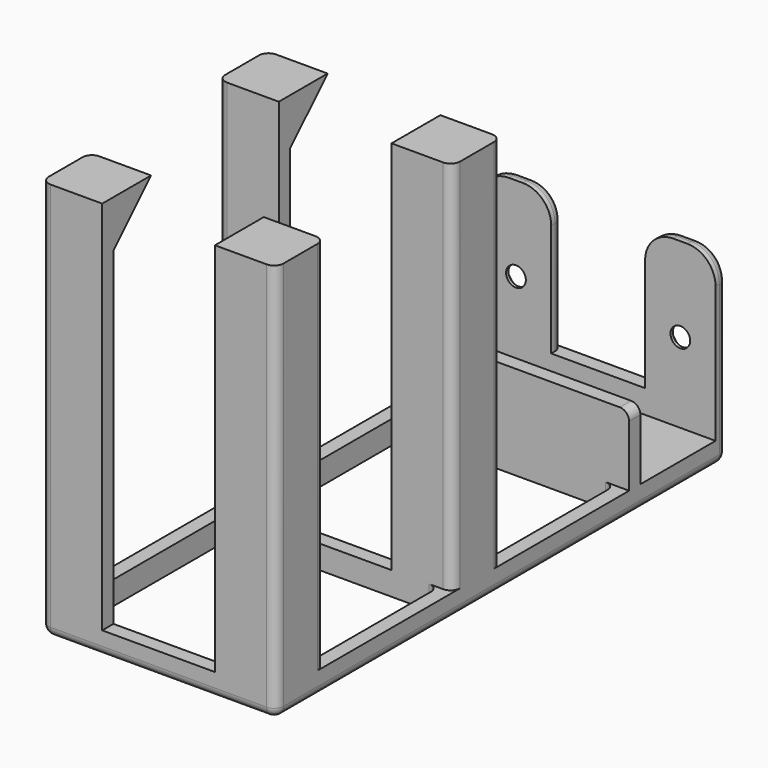
from build123d import *

# Parameters (mm, degrees)
F0_W            = 50
F0_H            = 120
F0_W_2          = 44
F0_H_2          = 44
F1_DEPTH        = 5
F2_W            = 50
F2_H            = 3
F3_DEPTH        = 35
F4_DEPTH        = 15
F5_DEPTH        = 80
F6_W            = 10
F6_H            = 10
F7_W            = 10
F7_H            = 10
F8_DEPTH        = 10
F9_SIZE         = 9.99999
F10_W           = 20
F10_H           = 30
F11_DEPTH       = 3
F12_R           = 6
F13_F1_R        = 2
F13_F2_R        = 2
F13_F3_R        = 2
F13_F4_R        = 2
F13_F5_R        = 2
F13_F6_R        = 2
F13_F7_R        = 2
F13_F8_R        = 2
F13_F9_R        = 2
F13_F10_R       = 2
F13_F11_R       = 2
F13_F12_R       = 2
F13_F13_R       = 2
F13_F14_R       = 2
F13_F15_R       = 2
F13_F16_R       = 2
F13_F17_R       = 2
F13_F18_R       = 2
F13_F19_R       = 2
F13_F20_R       = 2
F15_D           = 4.2
F15_DEPTH       = 12
F15_CSINK_D     = 8.96
F15_CSINK_ANGLE = 90
F15_TIP         = 1.2618073


# Not quite as in the source:
# - a fillet or chamfer is up to 0.001 mm smaller than in the source, because OpenCascade refuses the exact size


with BuildPart() as f1:
    # F0 (on Top) → F1 (new body)
    with BuildSketch(Plane.XY):
        with Locations((0, 11.5)):
            Rectangle(F0_W, F0_H)
        with Locations((0, -23.5)):
            Rectangle(F0_W_2, F0_H_2, mode=Mode.SUBTRACT)
        with Locations((0, 23.5)):
            Rectangle(F0_W_2, F0_H_2, mode=Mode.SUBTRACT)
    extrude(amount=F1_DEPTH)

    # F2 (on face) → F3 (join)
    with BuildSketch(Plane.XY.offset(5)):
        with Locations((0, 70)):
            Rectangle(F2_W, F2_H)
    extrude(amount=F3_DEPTH)

    # F2 (on face) → F4 (join)
    with BuildSketch(Plane.XY.offset(5)):
        Polygon((25, 48.5), (-25, 48.5), (-25, 45.5), (-22, 45.5), (22, 45.5), (25, 45.5), align=None)
    extrude(amount=F4_DEPTH)

    # F2 (on face) → F5 (join)
    with BuildSketch(Plane.XY.offset(5)):
        Polygon((-22, 11.5), (-25, 11.5), (-25, -1.5), (-22, -1.5), (-12, -1.5), (-12, 1.5), (-22, 1.5), align=None)
        Polygon((25, -1.5), (25, 11.5), (22, 11.5), (22, 1.5), (12, 1.5), (12, -1.5), (22, -1.5), align=None)
        Polygon((-22, -35.5), (-25, -35.5), (-25, -48.5), (-12, -48.5), (-12, -45.5), (-22, -45.5), align=None)
        Polygon((25, -48.5), (25, -35.5), (22, -35.5), (22, -45.5), (12, -45.5), (12, -48.5), align=None)
    extrude(amount=F5_DEPTH)

    # F6 (on face) + F7 (on face) → F8 (join)
    with BuildSketch(Plane(origin=(0, 1.5, 0), x_dir=(-1, 0, 0), z_dir=(0, 1, 0))):
        with Locations((-17, 80)):
            Rectangle(F6_W, F6_H)
        with Locations((17, 80)):
            Rectangle(F6_W, F6_H)
    with BuildSketch(Plane(origin=(0, -45.5, 0), x_dir=(-1, 0, 0), z_dir=(0, 1, 0))):
        with Locations((17, 80)):
            Rectangle(F7_W, F7_H)
        with Locations((-17, 80)):
            Rectangle(F7_W, F7_H)
    extrude(amount=F8_DEPTH)

    # F9 (size 10 in the source; OpenCascade refuses exactly that, so slightly less here)
    f9_edges = [f1.edges().sort_by_distance(p)[0] for p in [
        (-17, 11.5, 75),
        (-17, -35.5, 75),
        (17, 11.5, 75),
        (17, -35.5, 75),
    ]]
    chamfer(f9_edges, length=F9_SIZE)

    # F10 (on face) → F11 (cut, through all)
    with BuildSketch(Plane(origin=(0, 71.5, 0), x_dir=(-1, 0, 0), z_dir=(0, 1, 0))):
        with Locations((0, 25)):
            Rectangle(F10_W, F10_H)
    extrude(amount=-F11_DEPTH, mode=Mode.SUBTRACT)

    # F12
    f12_edges = [f1.edges().sort_by_distance(p)[0] for p in [
        (25, 70, 40),
        (10, 70, 40),
        (-10, 70, 40),
        (-25, 70, 40),
    ]]
    fillet(f12_edges, radius=F12_R)

    # F13: fillet of radius 2 on 36 edges, made by hand

    # F13_f1
    f13_f1_edges = [f1.edges().sort_by_distance(p)[0] for p in [
        (25, 71.5, 17),
        (23.2426406871, 71.5, 38.2426406871),
        (17.5, 71.5, 40),
        (11.7573593129, 71.5, 38.2426406871),
        (10, 71.5, 22),
    ]]
    fillet(f13_f1_edges, radius=F13_F1_R)

    # F13_f2
    f13_f2_edges = [f1.edges().sort_by_distance(p)[0] for p in [
        (25, 10.5, 0),
    ]]
    fillet(f13_f2_edges, radius=F13_F2_R)

    # F13_f3
    f13_f3_edges = [f1.edges().sort_by_distance(p)[0] for p in [
        (25, 47, 20),
    ]]
    fillet(f13_f3_edges, radius=F13_F3_R)

    # F13_f4
    f13_f4_edges = [f1.edges().sort_by_distance(p)[0] for p in [
        (25, -48.5, 43.5),
    ]]
    fillet(f13_f4_edges, radius=F13_F4_R)

    # F13_f5
    f13_f5_edges = [f1.edges().sort_by_distance(p)[0] for p in [
        (25, -35.5, 45),
    ]]
    fillet(f13_f5_edges, radius=F13_F5_R)

    # F13_f6
    f13_f6_edges = [f1.edges().sort_by_distance(p)[0] for p in [
        (25, 11.5, 45),
    ]]
    fillet(f13_f6_edges, radius=F13_F6_R)

    # F13_f7
    f13_f7_edges = [f1.edges().sort_by_distance(p)[0] for p in [
        (25, -1.5, 45),
    ]]
    fillet(f13_f7_edges, radius=F13_F7_R)

    # F13_f8
    f13_f8_edges = [f1.edges().sort_by_distance(p)[0] for p in [
        (-25, 71.5, 18),
        (-23.2426406871, 71.5, 38.2426406871),
        (-17.5, 71.5, 40),
        (-11.7573593129, 71.5, 38.2426406871),
        (-10, 71.5, 22),
    ]]
    fillet(f13_f8_edges, radius=F13_F8_R)

    # F13_f9
    f13_f9_edges = [f1.edges().sort_by_distance(p)[0] for p in [
        (-25, -35.5, 45),
    ]]
    fillet(f13_f9_edges, radius=F13_F9_R)

    # F13_f10
    f13_f10_edges = [f1.edges().sort_by_distance(p)[0] for p in [
        (-25, 47, 20),
    ]]
    fillet(f13_f10_edges, radius=F13_F10_R)

    # F13_f11
    f13_f11_edges = [f1.edges().sort_by_distance(p)[0] for p in [
        (-25, -1.5, 45),
    ]]
    fillet(f13_f11_edges, radius=F13_F11_R)

    # F13_f12
    f13_f12_edges = [f1.edges().sort_by_distance(p)[0] for p in [
        (-25, 11.5, 45),
    ]]
    fillet(f13_f12_edges, radius=F13_F12_R)

    # F13_f13
    f13_f13_edges = [f1.edges().sort_by_distance(p)[0] for p in [
        (-22, 45.5, 2.5),
    ]]
    fillet(f13_f13_edges, radius=F13_F13_R)

    # F13_f14
    f13_f14_edges = [f1.edges().sort_by_distance(p)[0] for p in [
        (22, 45.5, 2.5),
    ]]
    fillet(f13_f14_edges, radius=F13_F14_R)

    # F13_f15
    f13_f15_edges = [f1.edges().sort_by_distance(p)[0] for p in [
        (-22, -1.5, 2.5),
    ]]
    fillet(f13_f15_edges, radius=F13_F15_R)

    # F13_f16
    f13_f16_edges = [f1.edges().sort_by_distance(p)[0] for p in [
        (22, -1.5, 2.5),
    ]]
    fillet(f13_f16_edges, radius=F13_F16_R)

    # F13_f17
    f13_f17_edges = [f1.edges().sort_by_distance(p)[0] for p in [
        (-22, -45.5, 37.5),
    ]]
    fillet(f13_f17_edges, radius=F13_F17_R)

    # F13_f18
    f13_f18_edges = [f1.edges().sort_by_distance(p)[0] for p in [
        (22, -45.5, 37.5),
    ]]
    fillet(f13_f18_edges, radius=F13_F18_R)

    # F13_f19
    f13_f19_edges = [f1.edges().sort_by_distance(p)[0] for p in [
        (-22, 1.5, 37.5),
    ]]
    fillet(f13_f19_edges, radius=F13_F19_R)

    # F13_f20
    f13_f20_edges = [f1.edges().sort_by_distance(p)[0] for p in [
        (22, 1.5, 37.5),
    ]]
    fillet(f13_f20_edges, radius=F13_F20_R)

    # F15
    with Locations(Plane(origin=(0, 71.5, 0), x_dir=(-1, 0, 0), z_dir=(0, 1, 0))):
        with Locations((-17.5, 22), (17.5, 22)):
            CounterSinkHole(F15_D / 2, F15_CSINK_D / 2, depth=F15_DEPTH, counter_sink_angle=F15_CSINK_ANGLE)
            with Locations((0, 0, -(F15_DEPTH + F15_TIP / 2))):  # 118° drill point
                Cone(0, F15_D / 2, F15_TIP, mode=Mode.SUBTRACT)


solid = f1.part
